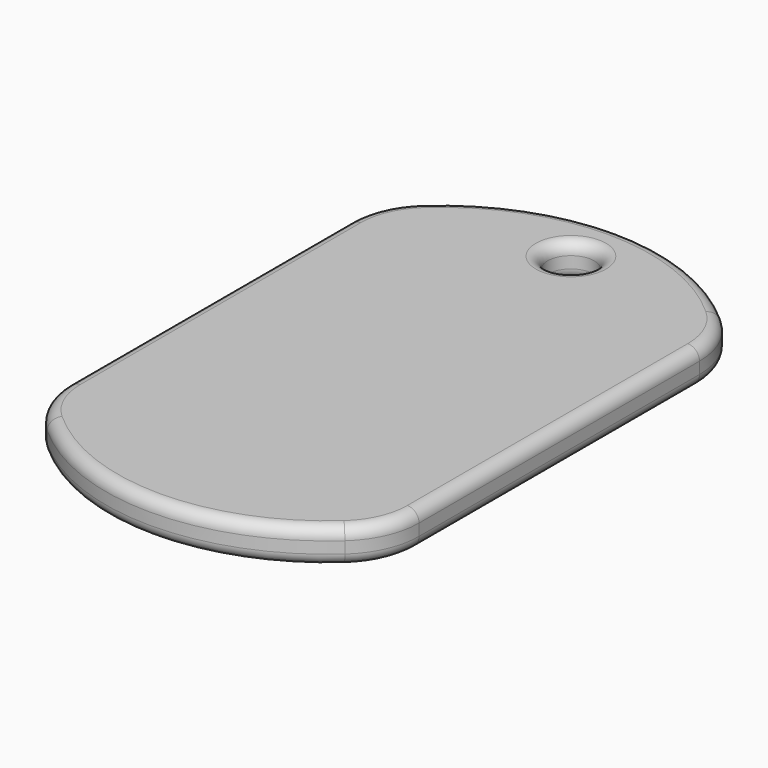
from build123d import *

# Parameters (mm, degrees)
F1_DEPTH = 3
F3_D     = 4
F4_R     = 1


# Not quite as in the source:
# - ends of sketch curves that miss each other by under 0.0002 mm in the source are joined


with BuildPart() as f1:
    # F0 (on Top) → F1 (new body)
    with BuildSketch(Plane.XY):
        with BuildLine():
            Line((15, -15), (15, 15.0000007931))
            ThreePointArc((15, 15.0000007931), (14.4074542357, 17.7922023165), (12.7319587629, 20.1030927835))
            ThreePointArc((12.7319587629, 20.1030927835), (0, 25), (-12.7319587629, 20.1030927835))
            ThreePointArc((-12.7319587629, 20.1030927835), (-14.4074543968, 17.7922019541), (-15, 15))
            Line((-15, 15), (-15, -15.0000007931))
            ThreePointArc((-15, -15.0000007931), (-14.4074543968, -17.7922019541), (-12.7319587629, -20.1030927835))
            ThreePointArc((-12.7319587629, -20.1030927835), (0, -25), (12.7319587629, -20.1030927835))
            ThreePointArc((12.7319587629, -20.1030927835), (14.4074542357, -17.7922023165), (15, -15))
        make_face()
    extrude(amount=F1_DEPTH)

    # F3 (through all)
    with Locations(Plane.XY.offset(3)):
        with Locations((0, 20)):
            Hole(F3_D / 2)

    # F4
    f4_edges = [f1.edges().sort_by_distance(p)[0] for p in [
        (14.407454, -17.792202, 3),
        (0, -25, 3),
        (15, 0, 3),
        (-14.407454, -17.792202, 3),
        (14.407454, 17.792202, 3),
        (-15, 0, 3),
        (0, 25, 3),
        (-14.407454, 17.792202, 3),
        (-2, 20, 3),
        (14.407454, -17.792202, 0),
        (0, -25, 0),
        (15, 0, 0),
        (-14.407454, -17.792202, 0),
        (14.407454, 17.792202, 0),
        (-15, 0, 0),
        (0, 25, 0),
        (-14.407454, 17.792202, 0),
        (-2, 20, 0),
    ]]
    fillet(f4_edges, radius=F4_R)


solid = f1.part
